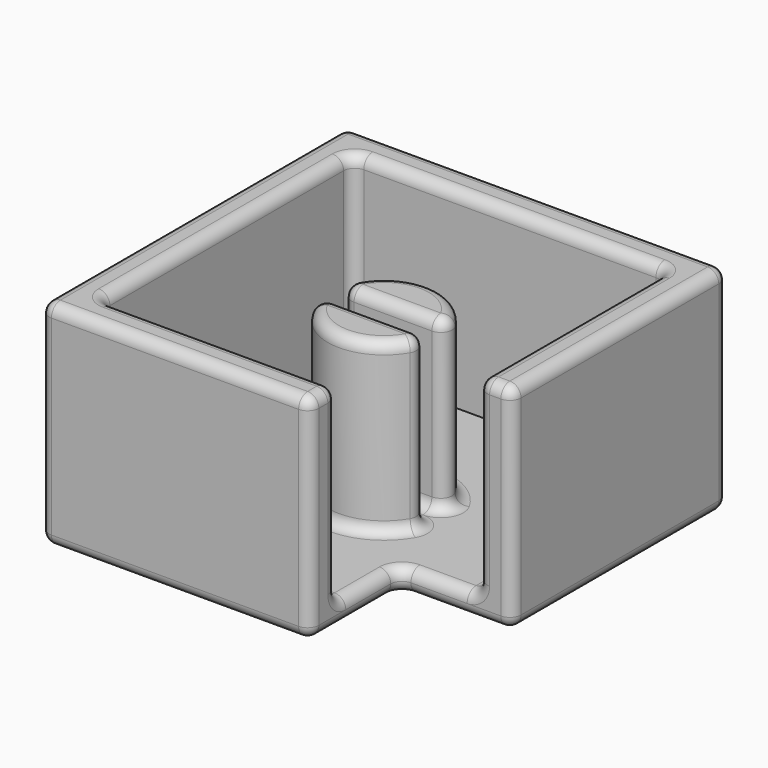
from build123d import *

# Parameters (mm, degrees)
F0_W     = 17
F0_H     = 17
F1_DEPTH = 1
F2_W     = 17
F2_H     = 17
F2_W_2   = 14
F2_H_2   = 14
F3_DEPTH = 8.5
F4_W     = 5
F4_H     = 9.5
F5_DEPTH = 5
F7_DEPTH = 7.5
F8_F1_R  = 0.5
F8_F2_R  = 0.4999
F9_R     = 0.49999


# Not quite as in the source:
# - a fillet or chamfer is up to 0.001 mm smaller than in the source, because OpenCascade refuses the exact size
# - a feature names something its author has since deleted; it is built from what else it names


with BuildPart() as f1:
    # F0 (on Top) → F1 (new body)
    with BuildSketch(Plane.XY):
        with Locations((-34.0035885349, 30.668237003)):
            Rectangle(F0_W, F0_H)
    extrude(amount=F1_DEPTH)

    # F2 (on face) → F3 (join)
    with BuildSketch(Plane.XY.offset(1)):
        with Locations((-34.0035885349, 30.668237003)):
            Rectangle(F2_W, F2_H)
        with Locations((-34.0035885349, 30.668237003)):
            Rectangle(F2_W_2, F2_H_2, mode=Mode.SUBTRACT)
    extrude(amount=F3_DEPTH)

    # F4 (on face) → F5 (cut)
    with BuildSketch(Plane.XZ.offset(-22.168237003)):
        with Locations((-28.0035885349, 4.75)):
            Rectangle(F4_W, F4_H)
    extrude(amount=-F5_DEPTH, mode=Mode.SUBTRACT)

    # F6 (on face) → F7 (join)
    with BuildSketch(Plane.XY.offset(1)):
        with BuildLine():
            Line((-31.5540987921, 30.168237003), (-36.4530782777, 30.168237003))
            ThreePointArc((-36.4530782777, 30.168237003), (-34.0035885349, 28.168237003), (-31.5540987921, 30.168237003))
        make_face()
        with BuildLine():
            Line((-36.4530782777, 31.168237003), (-31.5540987921, 31.168237003))
            ThreePointArc((-31.5540987921, 31.168237003), (-34.0035885349, 33.168237003), (-36.4530782777, 31.168237003))
        make_face()
    extrude(amount=F7_DEPTH)

    # F8: fillet of radius 0.5 on 31 edges, made by hand

    # F8_f1
    f8_f1_edges = [f1.edges().sort_by_distance(p)[0] for p in [
        (-35.7535885349, 23.668237003, 1),
        (-41.0035885349, 23.668237003, 5.25),
        (-41.0035885349, 30.668237003, 1),
        (-27.0035885349, 32.418237003, 1),
        (-27.0035885349, 37.668237003, 5.25),
        (-41.0035885349, 37.668237003, 5.25),
        (-30.5035885349, 27.168237003, 0.5),
    ]]
    fillet(f8_f1_edges, radius=F8_F1_R)

    # F8_f2 (radius 0.5 in the source; OpenCascade refuses exactly that, so slightly less here)
    f8_f2_edges = [f1.edges().sort_by_distance(p)[0] for p in [
        (-42.5035885349, 39.168237003, 4.75),
        (-42.5035885349, 22.168237003, 4.75),
        (-34.0035885349, 39.168237003, 9.5),
        (-42.5035885349, 30.668237003, 9.5),
        (-42.5035885349, 30.668237003, 0),
        (-34.0035885349, 39.168237003, 0),
        (-25.5035885349, 39.168237003, 4.75),
        (-34.0035885349, 37.668237003, 9.5),
        (-41.0035885349, 30.668237003, 9.5),
        (-35.5035885349, 23.668237003, 9.5),
        (-36.5035885349, 22.168237003, 9.5),
        (-30.5035885349, 22.918237003, 9.5),
        (-27.0035885349, 32.168237003, 9.5),
        (-25.5035885349, 33.168237003, 9.5),
        (-26.2535885349, 27.168237003, 9.5),
        (-27.0035885349, 27.168237003, 5.5),
        (-25.5035885349, 27.168237003, 4.75),
        (-36.5035885349, 22.168237003, 0),
        (-30.5035885349, 22.168237003, 4.75),
        (-30.5035885349, 24.418237003, 0),
        (-30.5035885349, 25.418237003, 1),
        (-27.7535885349, 27.168237003, 0),
        (-25.5035885349, 33.168237003, 0),
        (-30.5035885349, 23.668237003, 5.5),
        (-30.5035885349, 23.8146836124, 1.1464466094),
        (-30.3571419255, 27.0217903936, 0),
        (-30.3571419255, 27.0217903936, 1),
        (-27.1500351443, 27.168237003, 1.1464466094),
        (-27.1500351443, 37.5217903936, 9.5),
        (-40.8571419255, 23.8146836124, 9.5),
        (-40.8571419255, 37.5217903936, 9.5),
    ]]
    fillet(f8_f2_edges, radius=F8_F2_R)

    # F9 (radius 0.5 in the source; OpenCascade refuses exactly that, so slightly less here)
    f9_edges = [f1.edges().sort_by_distance(p)[0] for p in [
        (-34.003589, 33.168237, 8.5),
        (-34.003589, 31.168237, 8.5),
        (-34.003589, 30.168237, 8.5),
        (-34.003589, 28.168237, 8.5),
        (-31.554099, 31.168237, 4.75),
        (-36.453078, 30.168237, 4.75),
        (-34.003589, 28.168237, 1),
        (-36.453078, 31.168237, 4.75),
        (-34.003589, 33.168237, 1),
        (-34.003589, 30.168237, 1),
        (-34.003589, 31.168237, 1),
        (-31.554099, 30.168237, 4.75),
    ]]
    fillet(f9_edges, radius=F9_R)


solid = f1.part
